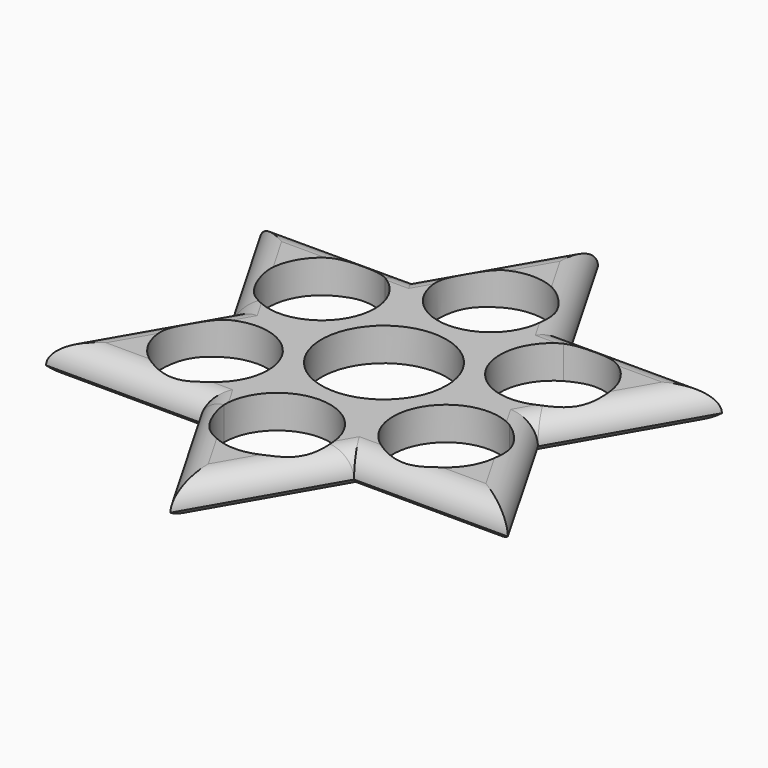
from build123d import *

# Parameters (mm, degrees)
F0_R          = 13.2
F1_DEPTH      = 7
F2_T4_DEPTH   = 57.5870860263
F2_T9_DEPTH   = 57.5217714755
F2_T14_DEPTH  = 57.5217714755
F2_T19_DEPTH  = 57.5870860263
F2_T24_DEPTH  = 57.5870860263
F2_T29_DEPTH  = 57.5217714755
F2_T34_DEPTH  = 57.5217714755
F2_T39_DEPTH  = 57.5870860263
F2_T44_DEPTH  = 57.5870860263
F2_T49_DEPTH  = 57.5217714755
F2_T54_DEPTH  = 57.5217714755
F2_T59_DEPTH  = 57.5870860263
F2_T65_DEPTH  = 57.5870860263
F2_S66_R      = 11.2
F2_T67_DEPTH  = 31
F2_S69_R      = 11.2
F2_T70_DEPTH  = 31
F2_T73_DEPTH  = 57.5870860263
F2_S74_R      = 11.2
F2_T75_DEPTH  = 33
F2_S77_R      = 11.2
F2_T78_DEPTH  = 33
F2_T84_DEPTH  = 57.5217714755
F2_S86_R      = 11.2
F2_T87_DEPTH  = 30
F2_S88_R      = 11.2
F2_T89_DEPTH  = 30
F2_T92_DEPTH  = 57.5217714755
F2_S94_R      = 11.2
F2_T95_DEPTH  = 33
F2_S96_R      = 11.2
F2_T97_DEPTH  = 33
F2_T103_DEPTH = 57.5870860263
F2_S105_R     = 11.2
F2_T106_DEPTH = 33
F2_S107_R     = 11.2
F2_T108_DEPTH = 33
F2_T111_DEPTH = 57.5870860263
F2_S113_R     = 11.2
F2_T114_DEPTH = 33
F2_S115_R     = 11.2
F2_T116_DEPTH = 33
F2_T122_DEPTH = 57.5217714755
F2_S124_R     = 11.2
F2_T125_DEPTH = 33
F2_S126_R     = 11.2
F2_T127_DEPTH = 33
F2_T130_DEPTH = 57.5217714755
F2_S132_R     = 11.2
F2_T133_DEPTH = 30
F2_S134_R     = 11.2
F2_T135_DEPTH = 30
F2_T141_DEPTH = 57.5870860263
F2_S143_R     = 11.2
F2_T144_DEPTH = 31
F2_S145_R     = 11.2
F2_T146_DEPTH = 31
F2_T149_DEPTH = 57.5870860263
F2_S151_R     = 11.2
F2_T152_DEPTH = 33
F2_S153_R     = 11.2
F2_T154_DEPTH = 33
F2_T160_DEPTH = 57.5217714755
F2_S161_R     = 11.2
F2_T162_DEPTH = 33
F2_S164_R     = 11.2
F2_T165_DEPTH = 33
F2_T168_DEPTH = 57.5217714755
F2_S169_R     = 11.2
F2_T170_DEPTH = 33
F2_S172_R     = 11.2
F2_T173_DEPTH = 33
F3_T4_DEPTH   = 52.5217714754
F3_T9_DEPTH   = 52.5870860261
F3_T14_DEPTH  = 52.5870860261
F3_T19_DEPTH  = 52.5217714754
F3_T24_DEPTH  = 52.5217714754
F3_T29_DEPTH  = 52.5870860261
F3_T34_DEPTH  = 52.5870860261
F3_T39_DEPTH  = 52.5217714754
F3_T44_DEPTH  = 52.5217714754
F3_T49_DEPTH  = 52.5870860261
F3_T54_DEPTH  = 52.5217714754
F3_T59_DEPTH  = 52.5870860261
F3_T65_DEPTH  = 52.5217714754
F3_T69_DEPTH  = 52.5217714754
F3_T76_DEPTH  = 52.5870860261
F3_T80_DEPTH  = 52.5870860261
F3_T87_DEPTH  = 52.5217714754
F3_T91_DEPTH  = 52.5217714754
F3_T98_DEPTH  = 52.5870860261
F3_T102_DEPTH = 52.5870860261
F3_T109_DEPTH = 52.5217714754
F3_T113_DEPTH = 52.5217714754
F3_T120_DEPTH = 52.5870860261
F3_T124_DEPTH = 52.5870860261


# Not quite as in the source:
# - a fillet or chamfer that OpenCascade refuses, or shapes differently, is made with other operations: its cross-section is extruded or revolved along the edge and cut away or added


with BuildPart() as f1:
    # F0 (on Top) → F1 (new body)
    with BuildSketch(Plane.XY):
        with BuildLine():
            Line((-16.2445816704, 28.1929764897), (-48.8316676967, 28.1929764897))
            Line((-48.8316676967, 28.1929764897), (-32.5707819589, 0.0282962158))
            Line((-32.5707819589, 0.0282962158), (-30.032715263, 4.4067698189))
            ThreePointArc((-30.032715263, 4.4067698189), (-34.1055736168, 19.7133328412), (-18.7990260705, 23.7862493557))
            Line((-18.7990260705, 23.7862493557), (-16.2445816704, 28.1929764897))
        make_face()
        with BuildLine():
            Line((0.0979717275, 56.3858678653), (-16.2445816704, 28.1929764897))
            Line((-16.2445816704, 28.1929764897), (-11.2, 28.1929764897))
            ThreePointArc((-11.2, 28.1929764897), (0, 39.3929764897), (11.2, 28.1929764897))
            Line((11.2, 28.1929764897), (16.3098962211, 28.1929764897))
            Line((16.3098962211, 28.1929764897), (0.0979717275, 56.3858678653))
        make_face()
        with BuildLine():
            Line((-11.2, 28.1929764897), (-16.2445816704, 28.1929764897))
            Line((-16.2445816704, 28.1929764897), (-18.7990260705, 23.7862493557))
            ThreePointArc((-18.7990260705, 23.7862493557), (-14.7114985514, 19.6880780406), (-13.2158338483, 14.0964882448))
            ThreePointArc((-13.2158338483, 14.0964882448), (-18.8242809265, 4.3921317014), (-30.032715263, 4.4067698189))
            Line((-30.032715263, 4.4067698189), (-32.5707819589, 0.0282962158))
            Line((-32.5707819589, 0.0282962158), (-30.0158338483, -4.3970037224))
            ThreePointArc((-30.0158338483, -4.3970037224), (-18.8158338483, -4.3970037224), (-13.2158338483, -14.0964882448))
            ThreePointArc((-13.2158338483, -14.0964882448), (-14.716349326, -19.6964882448), (-18.8158338483, -23.7959727672))
            Line((-18.8158338483, -23.7959727672), (-16.2935430131, -28.1647086453))
            Line((-16.2935430131, -28.1647086453), (-11.1999831676, -28.1735588213))
            ThreePointArc((-11.1999831676, -28.1735588213), (0.0097088378, -16.9929806978), (11.2, -28.1929764897))
            ThreePointArc((11.2, -28.1929764897), (11.1999957549, -28.2027278845), (11.1999830197, -28.2124792719))
            Line((11.1999830197, -28.2124792719), (16.2608857378, -28.2212727054))
            Line((16.2608857378, -28.2212727054), (18.8158338483, -23.7959727672))
            ThreePointArc((18.8158338483, -23.7959727672), (14.716349326, -8.4964882448), (30.0158338483, -4.3970037224))
            Line((30.0158338483, -4.3970037224), (32.5381246835, -0.0282678444))
            Line((32.5381246835, -0.0282678444), (29.9990092381, 4.3873094656))
            ThreePointArc((29.9990092381, 4.3873094656), (14.7066338546, 8.5133497474), (18.8327322433, 23.805709453))
            Line((18.8327322433, 23.805709453), (16.3098962211, 28.1929764897))
            Line((16.3098962211, 28.1929764897), (11.2, 28.1929764897))
            ThreePointArc((11.2, 28.1929764897), (0, 16.9929764897), (-11.2, 28.1929764897))
        make_face()
        Circle(F0_R, mode=Mode.SUBTRACT)
        with BuildLine():
            Line((-30.0158338483, -4.3970037224), (-32.5707819589, 0.0282962158))
            Line((-32.5707819589, 0.0282962158), (-48.8805798496, -28.1080879278))
            Line((-48.8805798496, -28.1080879278), (-16.2935430131, -28.1647086453))
            Line((-16.2935430131, -28.1647086453), (-18.8158338483, -23.7959727672))
            ThreePointArc((-18.8158338483, -23.7959727672), (-34.1153183707, -19.6964882448), (-30.0158338483, -4.3970037224))
        make_face()
        with BuildLine():
            Line((48.8316676967, 28.1929764897), (16.3098962211, 28.1929764897))
            Line((16.3098962211, 28.1929764897), (18.8327322433, 23.805709453))
            ThreePointArc((18.8327322433, 23.805709453), (30.0242766814, 23.7910933935), (35.6158338483, 14.0964882448))
            ThreePointArc((35.6158338483, 14.0964882448), (34.1104603075, 8.4880822487), (29.9990092381, 4.3873094656))
            Line((29.9990092381, 4.3873094656), (32.5381246835, -0.0282678444))
            Line((32.5381246835, -0.0282678444), (48.8316676967, 28.1929764897))
        make_face()
        with BuildLine():
            Line((-11.1999831676, -28.1735588213), (-16.2935430131, -28.1647086453))
            Line((-16.2935430131, -28.1647086453), (0, -56.3859529793))
            Line((0, -56.3859529793), (16.2608857378, -28.2212727054))
            Line((16.2608857378, -28.2212727054), (11.1999830197, -28.2124792719))
            ThreePointArc((11.1999830197, -28.2124792719), (-0.0194602253, -39.3929595834), (-11.1999831676, -28.1735588213))
        make_face()
        with BuildLine():
            Line((48.7826081221, -28.2777799376), (32.5381246835, -0.0282678444))
            Line((32.5381246835, -0.0282678444), (30.0158338483, -4.3970037224))
            ThreePointArc((30.0158338483, -4.3970037224), (34.1153183707, -8.4964882448), (35.6158338483, -14.0964882448))
            ThreePointArc((35.6158338483, -14.0964882448), (30.0158338483, -23.7959727672), (18.8158338483, -23.7959727672))
            Line((18.8158338483, -23.7959727672), (16.2608857378, -28.2212727054))
            Line((16.2608857378, -28.2212727054), (48.7826081221, -28.2777799376))
        make_face()
    extrude(amount=F1_DEPTH)

    # F2: fillet of radius 5 on 12 edges, made by hand


with BuildPart() as f2_tool2:
    # F2_s3 → F2_t4 (new body)
    with BuildSketch(Plane(origin=(30.7580755612, 53.0614196024, 0), x_dir=(0, 0, 1), z_dir=(-0.5015039818, -0.8651553365, 0))):
        with BuildLine():
            ThreePointArc((2, 28.1929764897), (5.5355339059, 26.7285103956), (7, 23.1929764897))
            Line((7, 23.1929764897), (7, 28.1929764897))
            Line((7, 28.1929764897), (2, 28.1929764897))
        make_face()
    extrude(amount=F2_T4_DEPTH)

    split(bisect_by=Plane.XZ.offset(-28.1929764897), keep=Keep.BOTTOM)


with BuildPart() as f1_1:
    add(f1.part)

    # F2_t1: cut F2_tool2
    add(f2_tool2.part, mode=Mode.SUBTRACT)


with BuildPart() as f2_tool7:
    # F2_s8 → F2_t9 (new body)
    with BuildSketch(Plane(origin=(-1.8992123449, 3.3027718184, 0), x_dir=(0, 0, 1), z_dir=(-0.4984945087, 0.8668928566, 0))):
        with BuildLine():
            ThreePointArc((2, 28.1929764897), (5.5355339059, 26.7285103956), (7, 23.1929764897))
            Line((7, 23.1929764897), (7, 28.1929764897))
            Line((7, 28.1929764897), (2, 28.1929764897))
        make_face()
    extrude(amount=F2_T9_DEPTH)

    split(bisect_by=Plane.XZ.offset(-28.1929764897), keep=Keep.BOTTOM)


with BuildPart() as f1_2:
    add(f1_1.part)

    # F2_t6: cut F2_tool7
    add(f2_tool7.part, mode=Mode.SUBTRACT)


with BuildPart() as f2_tool12:
    # F2_s13 → F2_t14 (new body)
    with BuildSketch(Plane.YZ.offset(61.3316676967)):
        with BuildLine():
            ThreePointArc((28.1929764897, 2), (26.7285103956, 5.5355339059), (23.1929764897, 7))
            Line((23.1929764897, 7), (28.1929764897, 7))
            Line((28.1929764897, 7), (28.1929764897, 2))
        make_face()
    extrude(amount=-F2_T14_DEPTH)

    split(bisect_by=Plane(origin=(24.4402899248, 14.0540439639, 0), x_dir=(0, 0, 1), z_dir=(0.8668928566, 0.4984945087, 0)), keep=Keep.TOP)


with BuildPart() as f1_3:
    add(f1_2.part)

    # F2_t11: cut F2_tool12
    add(f2_tool12.part, mode=Mode.SUBTRACT)


with BuildPart() as f2_tool17:
    # F2_s18 → F2_t19 (new body)
    with BuildSketch(Plane(origin=(1.8722908352, 3.2429028531, 0), x_dir=(0, 0, 1), z_dir=(0.5, 0.8660254038, 0))):
        with BuildLine():
            ThreePointArc((2, 28.1929764897), (5.5355339059, 26.7285103956), (7, 23.1929764897))
            Line((7, 23.1929764897), (7, 28.1929764897))
            Line((7, 28.1929764897), (2, 28.1929764897))
        make_face()
    extrude(amount=F2_T19_DEPTH)

    split(bisect_by=Plane(origin=(24.4402899248, 14.0540439639, 0), x_dir=(0, 0, 1), z_dir=(0.8668928566, 0.4984945087, 0)), keep=Keep.TOP)


with BuildPart() as f1_4:
    add(f1_3.part)

    # F2_t16: cut F2_tool17
    add(f2_tool17.part, mode=Mode.SUBTRACT)


with BuildPart() as f2_tool22:
    # F2_s23 → F2_t24 (new body)
    with BuildSketch(Plane(origin=(30.573499556, -53.1679846088, 0), x_dir=(0, 0, 1), z_dir=(-0.4984945087, 0.8668928566, 0))):
        with BuildLine():
            ThreePointArc((2, 28.1929764897), (5.5355339059, 26.7285103956), (7, 23.1929764897))
            Line((7, 23.1929764897), (7, 28.1929764897))
            Line((7, 28.1929764897), (2, 28.1929764897))
        make_face()
    extrude(amount=F2_T24_DEPTH)

    split(bisect_by=Plane(origin=(24.4158338483, -14.0964882448, 0), x_dir=(0, 0, 1), z_dir=(0.8660254038, -0.5, 0)), keep=Keep.TOP)


with BuildPart() as f1_5:
    add(f1_4.part)

    # F2_t21: cut F2_tool22
    add(f2_tool22.part, mode=Mode.SUBTRACT)


with BuildPart() as f2_tool27:
    # F2_s28 → F2_t29 (new body)
    with BuildSketch(Plane(origin=(3.8098904701, -0.0066197713, 0), x_dir=(0, 0, 1), z_dir=(0.9999984905, -0.0017375201, 0))):
        with BuildLine():
            ThreePointArc((2, 28.1929764897), (5.5355339059, 26.7285103956), (7, 23.1929764897))
            Line((7, 23.1929764897), (7, 28.1929764897))
            Line((7, 28.1929764897), (2, 28.1929764897))
        make_face()
    extrude(amount=F2_T29_DEPTH)

    split(bisect_by=Plane(origin=(24.4158338483, -14.0964882448, 0), x_dir=(0, 0, 1), z_dir=(0.8660254038, -0.5, 0)), keep=Keep.TOP)


with BuildPart() as f1_6:
    add(f1_5.part)

    # F2_t26: cut F2_tool27
    add(f2_tool27.part, mode=Mode.SUBTRACT)


with BuildPart() as f2_tool32:
    # F2_s33 → F2_t34 (new body)
    with BuildSketch(Plane(origin=(-30.6658338483, -53.1147822818, 0), x_dir=(0, 0, 1), z_dir=(0.5, 0.8660254038, 0))):
        with BuildLine():
            ThreePointArc((2, 28.1929764897), (5.5355339059, 26.7285103956), (7, 23.1929764897))
            Line((7, 23.1929764897), (7, 28.1929764897))
            Line((7, 28.1929764897), (2, 28.1929764897))
        make_face()
    extrude(amount=F2_T34_DEPTH)

    split(bisect_by=Plane(origin=(-0.0489858638, -28.1929339327, 0), x_dir=(0, 0, 1), z_dir=(-0.0017375201, -0.9999984905, 0)), keep=Keep.TOP)


with BuildPart() as f1_7:
    add(f1_6.part)

    # F2_t31: cut F2_tool32
    add(f2_tool32.part, mode=Mode.SUBTRACT)


with BuildPart() as f2_tool37:
    # F2_s38 → F2_t39 (new body)
    with BuildSketch(Plane(origin=(1.8722908352, -3.2429028531, 0), x_dir=(0, 0, 1), z_dir=(0.5, -0.8660254038, 0))):
        with BuildLine():
            ThreePointArc((2, 28.1929764897), (5.5355339059, 26.7285103956), (7, 23.1929764897))
            Line((7, 23.1929764897), (7, 28.1929764897))
            Line((7, 28.1929764897), (2, 28.1929764897))
        make_face()
    extrude(amount=F2_T39_DEPTH)

    split(bisect_by=Plane(origin=(-0.0489858638, -28.1929339327, 0), x_dir=(0, 0, 1), z_dir=(-0.0017375201, -0.9999984905, 0)), keep=Keep.TOP)


with BuildPart() as f1_8:
    add(f1_7.part)

    # F2_t36: cut F2_tool37
    add(f2_tool37.part, mode=Mode.SUBTRACT)


with BuildPart() as f2_tool42:
    # F2_s43 → F2_t44 (new body)
    with BuildSketch(Plane(origin=(-61.3315751172, 0.1065650063, 0), x_dir=(0, 0, 1), z_dir=(0.9999984905, -0.0017375201, 0))):
        with BuildLine():
            ThreePointArc((2, 28.1929764897), (5.5355339059, 26.7285103956), (7, 23.1929764897))
            Line((7, 23.1929764897), (7, 28.1929764897))
            Line((7, 28.1929764897), (2, 28.1929764897))
        make_face()
    extrude(amount=F2_T44_DEPTH)

    split(bisect_by=Plane(origin=(-24.4158338483, -14.0964882448, 0), x_dir=(0, 0, 1), z_dir=(-0.8660254038, -0.5, 0)), keep=Keep.TOP)


with BuildPart() as f1_9:
    add(f1_8.part)

    # F2_t41: cut F2_tool42
    add(f2_tool42.part, mode=Mode.SUBTRACT)


with BuildPart() as f2_tool47:
    # F2_s48 → F2_t49 (new body)
    with BuildSketch(Plane(origin=(-1.9106781252, -3.2961520471, 0), x_dir=(0, 0, 1), z_dir=(-0.5015039818, -0.8651553365, 0))):
        with BuildLine():
            ThreePointArc((2, 28.1929764897), (5.5355339059, 26.7285103956), (7, 23.1929764897))
            Line((7, 23.1929764897), (7, 28.1929764897))
            Line((7, 28.1929764897), (2, 28.1929764897))
        make_face()
    extrude(amount=F2_T49_DEPTH)

    split(bisect_by=Plane(origin=(-24.4158338483, -14.0964882448, 0), x_dir=(0, 0, 1), z_dir=(-0.8660254038, -0.5, 0)), keep=Keep.TOP)


with BuildPart() as f1_10:
    add(f1_9.part)

    # F2_t46: cut F2_tool47
    add(f2_tool47.part, mode=Mode.SUBTRACT)


with BuildPart() as f2_tool52:
    # F2_s53 → F2_t54 (new body)
    with BuildSketch(Plane(origin=(-30.6658338483, 53.1147822818, 0), x_dir=(0, 0, 1), z_dir=(0.5, -0.8660254038, 0))):
        with BuildLine():
            ThreePointArc((2, 28.1929764897), (5.5355339059, 26.7285103956), (7, 23.1929764897))
            Line((7, 23.1929764897), (7, 28.1929764897))
            Line((7, 28.1929764897), (2, 28.1929764897))
        make_face()
    extrude(amount=F2_T54_DEPTH)

    split(bisect_by=Plane(origin=(-24.391304061, 14.1388899688, 0), x_dir=(0, 0, 1), z_dir=(-0.8651553365, 0.5015039818, 0)), keep=Keep.TOP)


with BuildPart() as f1_11:
    add(f1_10.part)

    # F2_t51: cut F2_tool52
    add(f2_tool52.part, mode=Mode.SUBTRACT)


with BuildPart() as f2_tool57:
    # F2_s58 → F2_t59 (new body)
    with BuildSketch(Plane.YZ.offset(-3.7445816704)):
        with BuildLine():
            ThreePointArc((28.1929764897, 2), (26.7285103956, 5.5355339059), (23.1929764897, 7))
            Line((23.1929764897, 7), (28.1929764897, 7))
            Line((28.1929764897, 7), (28.1929764897, 2))
        make_face()
    extrude(amount=-F2_T59_DEPTH)

    split(bisect_by=Plane(origin=(-24.391304061, 14.1388899688, 0), x_dir=(0, 0, 1), z_dir=(-0.8651553365, 0.5015039818, 0)), keep=Keep.TOP)


with BuildPart() as f1_12:
    add(f1_11.part)

    # F2_t56: cut F2_tool57
    add(f2_tool57.part, mode=Mode.SUBTRACT)


with BuildPart() as f2_tool63:
    # F2_s64 → F2_t65 (new body)
    with BuildSketch(Plane.YZ.offset(-3.7445816704)):
        with BuildLine():
            ThreePointArc((28.1929764897, 2), (26.7285103956, 5.5355339059), (23.1929764897, 7))
            Line((23.1929764897, 7), (28.1929764897, 7))
            Line((28.1929764897, 7), (28.1929764897, 2))
        make_face()
    extrude(amount=-F2_T65_DEPTH)

    # F2_s66 → F2_t67 (cut, symmetric)
    with BuildSketch(Plane.XY.offset(4.5)):
        with Locations((-24.4158338483, 14.0964882448)):
            Circle(F2_S66_R)
    extrude(amount=F2_T67_DEPTH, both=True, mode=Mode.SUBTRACT)

    split(bisect_by=Plane(origin=(-24.391304061, 14.1388899688, 0), x_dir=(0, 0, 1), z_dir=(0.8651553365, -0.5015039818, 0)), keep=Keep.TOP)

    # F2_s69 → F2_t70 (cut, symmetric)
    with BuildSketch(Plane.XY.offset(4.5)):
        with Locations((0, 28.1929764897)):
            Circle(F2_S69_R)
    extrude(amount=F2_T70_DEPTH, both=True, mode=Mode.SUBTRACT)


with BuildPart() as f2_tool71:
    # F2_s72 → F2_t73 (new body)
    with BuildSketch(Plane(origin=(30.7580755612, 53.0614196024, 0), x_dir=(0, 0, 1), z_dir=(-0.5015039818, -0.8651553365, 0))):
        with BuildLine():
            ThreePointArc((2, 28.1929764897), (5.5355339059, 26.7285103956), (7, 23.1929764897))
            Line((7, 23.1929764897), (7, 28.1929764897))
            Line((7, 28.1929764897), (2, 28.1929764897))
        make_face()
    extrude(amount=F2_T73_DEPTH)

    # F2_s74 → F2_t75 (cut, symmetric)
    with BuildSketch(Plane.XY.offset(4.5)):
        with Locations((-24.4158338483, 14.0964882448)):
            Circle(F2_S74_R)
    extrude(amount=F2_T75_DEPTH, both=True, mode=Mode.SUBTRACT)

    split(bisect_by=Plane.XZ.offset(-28.1929764897), keep=Keep.TOP)

    # F2_s77 → F2_t78 (cut, symmetric)
    with BuildSketch(Plane.XY.offset(4.5)):
        with Locations((0, 28.1929764897)):
            Circle(F2_S77_R)
    extrude(amount=F2_T78_DEPTH, both=True, mode=Mode.SUBTRACT)


with BuildPart() as f2_tool63_1:
    add(f2_tool63.part)

    # F2_t79: intersect F2_tool71
    add(f2_tool71.part, mode=Mode.INTERSECT)


with BuildPart() as f1_13:
    add(f1_12.part)

    # F2_t61: cut F2_tool63
    add(f2_tool63_1.part, mode=Mode.SUBTRACT)


with BuildPart() as f2_tool82:
    # F2_s83 → F2_t84 (new body)
    with BuildSketch(Plane.YZ.offset(61.3316676967)):
        with BuildLine():
            ThreePointArc((28.1929764897, 2), (26.7285103956, 5.5355339059), (23.1929764897, 7))
            Line((23.1929764897, 7), (28.1929764897, 7))
            Line((28.1929764897, 7), (28.1929764897, 2))
        make_face()
    extrude(amount=-F2_T84_DEPTH)

    split(bisect_by=Plane(origin=(24.4402899248, 14.0540439639, 0), x_dir=(0, 0, 1), z_dir=(-0.8668928566, -0.4984945087, 0)), keep=Keep.TOP)

    # F2_s86 → F2_t87 (cut, symmetric)
    with BuildSketch(Plane.XY.offset(4.5)):
        with Locations((24.4158338483, 14.0964882448)):
            Circle(F2_S86_R)
    extrude(amount=F2_T87_DEPTH, both=True, mode=Mode.SUBTRACT)

    # F2_s88 → F2_t89 (cut, symmetric)
    with BuildSketch(Plane.XY.offset(4.5)):
        with Locations((0, 28.1929764897)):
            Circle(F2_S88_R)
    extrude(amount=F2_T89_DEPTH, both=True, mode=Mode.SUBTRACT)


with BuildPart() as f2_tool90:
    # F2_s91 → F2_t92 (new body)
    with BuildSketch(Plane(origin=(-1.8992123449, 3.3027718184, 0), x_dir=(0, 0, 1), z_dir=(-0.4984945087, 0.8668928566, 0))):
        with BuildLine():
            ThreePointArc((2, 28.1929764897), (5.5355339059, 26.7285103956), (7, 23.1929764897))
            Line((7, 23.1929764897), (7, 28.1929764897))
            Line((7, 28.1929764897), (2, 28.1929764897))
        make_face()
    extrude(amount=F2_T92_DEPTH)

    split(bisect_by=Plane.XZ.offset(-28.1929764897), keep=Keep.TOP)

    # F2_s94 → F2_t95 (cut, symmetric)
    with BuildSketch(Plane.XY.offset(4.5)):
        with Locations((24.4158338483, 14.0964882448)):
            Circle(F2_S94_R)
    extrude(amount=F2_T95_DEPTH, both=True, mode=Mode.SUBTRACT)

    # F2_s96 → F2_t97 (cut, symmetric)
    with BuildSketch(Plane.XY.offset(4.5)):
        with Locations((0, 28.1929764897)):
            Circle(F2_S96_R)
    extrude(amount=F2_T97_DEPTH, both=True, mode=Mode.SUBTRACT)


with BuildPart() as f2_tool82_1:
    add(f2_tool82.part)

    # F2_t98: intersect F2_tool90
    add(f2_tool90.part, mode=Mode.INTERSECT)


with BuildPart() as f1_14:
    add(f1_13.part)

    # F2_t80: cut F2_tool82
    add(f2_tool82_1.part, mode=Mode.SUBTRACT)


with BuildPart() as f2_tool101:
    # F2_s102 → F2_t103 (new body)
    with BuildSketch(Plane(origin=(30.573499556, -53.1679846088, 0), x_dir=(0, 0, 1), z_dir=(-0.4984945087, 0.8668928566, 0))):
        with BuildLine():
            ThreePointArc((2, 28.1929764897), (5.5355339059, 26.7285103956), (7, 23.1929764897))
            Line((7, 23.1929764897), (7, 28.1929764897))
            Line((7, 28.1929764897), (2, 28.1929764897))
        make_face()
    extrude(amount=F2_T103_DEPTH)

    split(bisect_by=Plane(origin=(24.4158338483, -14.0964882448, 0), x_dir=(0, 0, 1), z_dir=(-0.8660254038, 0.5, 0)), keep=Keep.TOP)

    # F2_s105 → F2_t106 (cut, symmetric)
    with BuildSketch(Plane.XY.offset(4.5)):
        with Locations((24.4158338483, -14.0964882448)):
            Circle(F2_S105_R)
    extrude(amount=F2_T106_DEPTH, both=True, mode=Mode.SUBTRACT)

    # F2_s107 → F2_t108 (cut, symmetric)
    with BuildSketch(Plane.XY.offset(4.5)):
        with Locations((24.4158338483, 14.0964882448)):
            Circle(F2_S107_R)
    extrude(amount=F2_T108_DEPTH, both=True, mode=Mode.SUBTRACT)


with BuildPart() as f2_tool109:
    # F2_s110 → F2_t111 (new body)
    with BuildSketch(Plane(origin=(1.8722908352, 3.2429028531, 0), x_dir=(0, 0, 1), z_dir=(0.5, 0.8660254038, 0))):
        with BuildLine():
            ThreePointArc((2, 28.1929764897), (5.5355339059, 26.7285103956), (7, 23.1929764897))
            Line((7, 23.1929764897), (7, 28.1929764897))
            Line((7, 28.1929764897), (2, 28.1929764897))
        make_face()
    extrude(amount=F2_T111_DEPTH)

    split(bisect_by=Plane(origin=(24.4402899248, 14.0540439639, 0), x_dir=(0, 0, 1), z_dir=(-0.8668928566, -0.4984945087, 0)), keep=Keep.TOP)

    # F2_s113 → F2_t114 (cut, symmetric)
    with BuildSketch(Plane.XY.offset(4.5)):
        with Locations((24.4158338483, -14.0964882448)):
            Circle(F2_S113_R)
    extrude(amount=F2_T114_DEPTH, both=True, mode=Mode.SUBTRACT)

    # F2_s115 → F2_t116 (cut, symmetric)
    with BuildSketch(Plane.XY.offset(4.5)):
        with Locations((24.4158338483, 14.0964882448)):
            Circle(F2_S115_R)
    extrude(amount=F2_T116_DEPTH, both=True, mode=Mode.SUBTRACT)


with BuildPart() as f2_tool101_1:
    add(f2_tool101.part)

    # F2_t117: intersect F2_tool109
    add(f2_tool109.part, mode=Mode.INTERSECT)


with BuildPart() as f1_15:
    add(f1_14.part)

    # F2_t99: cut F2_tool101
    add(f2_tool101_1.part, mode=Mode.SUBTRACT)


with BuildPart() as f2_tool120:
    # F2_s121 → F2_t122 (new body)
    with BuildSketch(Plane(origin=(-30.6658338483, -53.1147822818, 0), x_dir=(0, 0, 1), z_dir=(0.5, 0.8660254038, 0))):
        with BuildLine():
            ThreePointArc((2, 28.1929764897), (5.5355339059, 26.7285103956), (7, 23.1929764897))
            Line((7, 23.1929764897), (7, 28.1929764897))
            Line((7, 28.1929764897), (2, 28.1929764897))
        make_face()
    extrude(amount=F2_T122_DEPTH)

    split(bisect_by=Plane(origin=(-0.0489858638, -28.1929339327, 0), x_dir=(0, 0, 1), z_dir=(0.0017375201, 0.9999984905, 0)), keep=Keep.TOP)

    # F2_s124 → F2_t125 (cut, symmetric)
    with BuildSketch(Plane.XY.offset(4.5)):
        with Locations((24.4158338483, -14.0964882448)):
            Circle(F2_S124_R)
    extrude(amount=F2_T125_DEPTH, both=True, mode=Mode.SUBTRACT)

    # F2_s126 → F2_t127 (cut, symmetric)
    with BuildSketch(Plane.XY.offset(4.5)):
        with Locations((0, -28.1929764897)):
            Circle(F2_S126_R)
    extrude(amount=F2_T127_DEPTH, both=True, mode=Mode.SUBTRACT)


with BuildPart() as f2_tool128:
    # F2_s129 → F2_t130 (new body)
    with BuildSketch(Plane(origin=(3.8098904701, -0.0066197713, 0), x_dir=(0, 0, 1), z_dir=(0.9999984905, -0.0017375201, 0))):
        with BuildLine():
            ThreePointArc((2, 28.1929764897), (5.5355339059, 26.7285103956), (7, 23.1929764897))
            Line((7, 23.1929764897), (7, 28.1929764897))
            Line((7, 28.1929764897), (2, 28.1929764897))
        make_face()
    extrude(amount=F2_T130_DEPTH)

    split(bisect_by=Plane(origin=(24.4158338483, -14.0964882448, 0), x_dir=(0, 0, 1), z_dir=(-0.8660254038, 0.5, 0)), keep=Keep.TOP)

    # F2_s132 → F2_t133 (cut, symmetric)
    with BuildSketch(Plane.XY.offset(4.5)):
        with Locations((24.4158338483, -14.0964882448)):
            Circle(F2_S132_R)
    extrude(amount=F2_T133_DEPTH, both=True, mode=Mode.SUBTRACT)

    # F2_s134 → F2_t135 (cut, symmetric)
    with BuildSketch(Plane.XY.offset(4.5)):
        with Locations((0, -28.1929764897)):
            Circle(F2_S134_R)
    extrude(amount=F2_T135_DEPTH, both=True, mode=Mode.SUBTRACT)


with BuildPart() as f2_tool120_1:
    add(f2_tool120.part)

    # F2_t136: intersect F2_tool128
    add(f2_tool128.part, mode=Mode.INTERSECT)


with BuildPart() as f1_16:
    add(f1_15.part)

    # F2_t118: cut F2_tool120
    add(f2_tool120_1.part, mode=Mode.SUBTRACT)


with BuildPart() as f2_tool139:
    # F2_s140 → F2_t141 (new body)
    with BuildSketch(Plane(origin=(-61.3315751172, 0.1065650063, 0), x_dir=(0, 0, 1), z_dir=(0.9999984905, -0.0017375201, 0))):
        with BuildLine():
            ThreePointArc((2, 28.1929764897), (5.5355339059, 26.7285103956), (7, 23.1929764897))
            Line((7, 23.1929764897), (7, 28.1929764897))
            Line((7, 28.1929764897), (2, 28.1929764897))
        make_face()
    extrude(amount=F2_T141_DEPTH)

    split(bisect_by=Plane(origin=(-24.4158338483, -14.0964882448, 0), x_dir=(0, 0, 1), z_dir=(0.8660254038, 0.5, 0)), keep=Keep.TOP)

    # F2_s143 → F2_t144 (cut, symmetric)
    with BuildSketch(Plane.XY.offset(4.5)):
        with Locations((0, -28.1929764897)):
            Circle(F2_S143_R)
    extrude(amount=F2_T144_DEPTH, both=True, mode=Mode.SUBTRACT)

    # F2_s145 → F2_t146 (cut, symmetric)
    with BuildSketch(Plane.XY.offset(4.5)):
        with Locations((-24.4158338483, -14.0964882448)):
            Circle(F2_S145_R)
    extrude(amount=F2_T146_DEPTH, both=True, mode=Mode.SUBTRACT)


with BuildPart() as f2_tool147:
    # F2_s148 → F2_t149 (new body)
    with BuildSketch(Plane(origin=(1.8722908352, -3.2429028531, 0), x_dir=(0, 0, 1), z_dir=(0.5, -0.8660254038, 0))):
        with BuildLine():
            ThreePointArc((2, 28.1929764897), (5.5355339059, 26.7285103956), (7, 23.1929764897))
            Line((7, 23.1929764897), (7, 28.1929764897))
            Line((7, 28.1929764897), (2, 28.1929764897))
        make_face()
    extrude(amount=F2_T149_DEPTH)

    split(bisect_by=Plane(origin=(-0.0489858638, -28.1929339327, 0), x_dir=(0, 0, 1), z_dir=(0.0017375201, 0.9999984905, 0)), keep=Keep.TOP)

    # F2_s151 → F2_t152 (cut, symmetric)
    with BuildSketch(Plane.XY.offset(4.5)):
        with Locations((0, -28.1929764897)):
            Circle(F2_S151_R)
    extrude(amount=F2_T152_DEPTH, both=True, mode=Mode.SUBTRACT)

    # F2_s153 → F2_t154 (cut, symmetric)
    with BuildSketch(Plane.XY.offset(4.5)):
        with Locations((-24.4158338483, -14.0964882448)):
            Circle(F2_S153_R)
    extrude(amount=F2_T154_DEPTH, both=True, mode=Mode.SUBTRACT)


with BuildPart() as f2_tool139_1:
    add(f2_tool139.part)

    # F2_t155: intersect F2_tool147
    add(f2_tool147.part, mode=Mode.INTERSECT)


with BuildPart() as f1_17:
    add(f1_16.part)

    # F2_t137: cut F2_tool139
    add(f2_tool139_1.part, mode=Mode.SUBTRACT)


with BuildPart() as f2_tool158:
    # F2_s159 → F2_t160 (new body)
    with BuildSketch(Plane(origin=(-30.6658338483, 53.1147822818, 0), x_dir=(0, 0, 1), z_dir=(0.5, -0.8660254038, 0))):
        with BuildLine():
            ThreePointArc((2, 28.1929764897), (5.5355339059, 26.7285103956), (7, 23.1929764897))
            Line((7, 23.1929764897), (7, 28.1929764897))
            Line((7, 28.1929764897), (2, 28.1929764897))
        make_face()
    extrude(amount=F2_T160_DEPTH)

    # F2_s161 → F2_t162 (cut, symmetric)
    with BuildSketch(Plane.XY.offset(4.5)):
        with Locations((-24.4158338483, 14.0964882448)):
            Circle(F2_S161_R)
    extrude(amount=F2_T162_DEPTH, both=True, mode=Mode.SUBTRACT)

    split(bisect_by=Plane(origin=(-24.391304061, 14.1388899688, 0), x_dir=(0, 0, 1), z_dir=(0.8651553365, -0.5015039818, 0)), keep=Keep.TOP)

    # F2_s164 → F2_t165 (cut, symmetric)
    with BuildSketch(Plane.XY.offset(4.5)):
        with Locations((-24.4158338483, -14.0964882448)):
            Circle(F2_S164_R)
    extrude(amount=F2_T165_DEPTH, both=True, mode=Mode.SUBTRACT)


with BuildPart() as f2_tool166:
    # F2_s167 → F2_t168 (new body)
    with BuildSketch(Plane(origin=(-1.9106781252, -3.2961520471, 0), x_dir=(0, 0, 1), z_dir=(-0.5015039818, -0.8651553365, 0))):
        with BuildLine():
            ThreePointArc((2, 28.1929764897), (5.5355339059, 26.7285103956), (7, 23.1929764897))
            Line((7, 23.1929764897), (7, 28.1929764897))
            Line((7, 28.1929764897), (2, 28.1929764897))
        make_face()
    extrude(amount=F2_T168_DEPTH)

    # F2_s169 → F2_t170 (cut, symmetric)
    with BuildSketch(Plane.XY.offset(4.5)):
        with Locations((-24.4158338483, 14.0964882448)):
            Circle(F2_S169_R)
    extrude(amount=F2_T170_DEPTH, both=True, mode=Mode.SUBTRACT)

    split(bisect_by=Plane(origin=(-24.4158338483, -14.0964882448, 0), x_dir=(0, 0, 1), z_dir=(0.8660254038, 0.5, 0)), keep=Keep.TOP)

    # F2_s172 → F2_t173 (cut, symmetric)
    with BuildSketch(Plane.XY.offset(4.5)):
        with Locations((-24.4158338483, -14.0964882448)):
            Circle(F2_S172_R)
    extrude(amount=F2_T173_DEPTH, both=True, mode=Mode.SUBTRACT)


with BuildPart() as f2_tool158_1:
    add(f2_tool158.part)

    # F2_t174: intersect F2_tool166
    add(f2_tool166.part, mode=Mode.INTERSECT)


with BuildPart() as f1_18:
    add(f1_17.part)

    # F2_t156: cut F2_tool158
    add(f2_tool158_1.part, mode=Mode.SUBTRACT)

    # F3: fillet of radius 5 on 12 edges, made by hand


with BuildPart() as f3_tool2:
    # F3_s3 → F3_t4 (new body)
    with BuildSketch(Plane.YZ.offset(58.8316676966)):
        with BuildLine():
            ThreePointArc((24.1929764897, 0), (26.4290444672, 0.527864045), (28.1929764897, 2))
            Line((28.1929764897, 2), (28.2729764897, 1.94))
            ThreePointArc((28.2729764897, 1.94), (28.2929764897, 1), (28.2929764897, 0))
            Line((28.2929764897, 0), (28.1929764897, -0.1))
            Line((28.1929764897, -0.1), (24.1929764897, -0.1))
            Line((24.1929764897, -0.1), (24.1929764897, 0))
        make_face()
    extrude(amount=-F3_T4_DEPTH)

    split(bisect_by=Plane(origin=(24.4402899248, 14.0540439639, 0), x_dir=(0, 0, 1), z_dir=(0.8668928566, 0.4984945087, 0)), keep=Keep.TOP)


with BuildPart() as f1_19:
    add(f1_18.part)

    # F3_t1: cut F3_tool2
    add(f3_tool2.part, mode=Mode.SUBTRACT)


with BuildPart() as f3_tool7:
    # F3_s8 → F3_t9 (new body)
    with BuildSketch(Plane(origin=(3.1222908352, 5.4079663627, 0), x_dir=(0, 0, 1), z_dir=(0.5, 0.8660254038, 0))):
        with BuildLine():
            ThreePointArc((0, 24.1929764897), (0.527864045, 26.4290444672), (2, 28.1929764897))
            Line((2, 28.1929764897), (1.94, 28.2729764897))
            ThreePointArc((1.94, 28.2729764897), (1, 28.2929764897), (0, 28.2929764897))
            Line((0, 28.2929764897), (-0.1, 28.1929764897))
            Line((-0.1, 28.1929764897), (-0.1, 24.1929764897))
            Line((-0.1, 24.1929764897), (0, 24.1929764897))
        make_face()
    extrude(amount=F3_T9_DEPTH)

    split(bisect_by=Plane(origin=(24.4402899248, 14.0540439639, 0), x_dir=(0, 0, 1), z_dir=(0.8668928566, 0.4984945087, 0)), keep=Keep.TOP)


with BuildPart() as f1_20:
    add(f1_19.part)

    # F3_t6: cut F3_tool7
    add(f3_tool7.part, mode=Mode.SUBTRACT)


with BuildPart() as f3_tool12:
    # F3_s13 → F3_t14 (new body)
    with BuildSketch(Plane(origin=(29.3272632842, -51.0007524672, 0), x_dir=(0, 0, 1), z_dir=(-0.4984945087, 0.8668928566, 0))):
        with BuildLine():
            ThreePointArc((0, 24.1929764897), (0.527864045, 26.4290444672), (2, 28.1929764897))
            Line((2, 28.1929764897), (1.94, 28.2729764897))
            ThreePointArc((1.94, 28.2729764897), (1, 28.2929764897), (0, 28.2929764897))
            Line((0, 28.2929764897), (-0.1, 28.1929764897))
            Line((-0.1, 28.1929764897), (-0.1, 24.1929764897))
            Line((-0.1, 24.1929764897), (0, 24.1929764897))
        make_face()
    extrude(amount=F3_T14_DEPTH)

    split(bisect_by=Plane(origin=(24.4158338483, -14.0964882448, 0), x_dir=(0, 0, 1), z_dir=(0.8660254038, -0.5, 0)), keep=Keep.TOP)


with BuildPart() as f1_21:
    add(f1_20.part)

    # F3_t11: cut F3_tool12
    add(f3_tool12.part, mode=Mode.SUBTRACT)


with BuildPart() as f3_tool17:
    # F3_s18 → F3_t19 (new body)
    with BuildSketch(Plane(origin=(6.3098866965, -0.0109635716, 0), x_dir=(0, 0, 1), z_dir=(0.9999984905, -0.0017375201, 0))):
        with BuildLine():
            ThreePointArc((0, 24.1929764897), (0.527864045, 26.4290444672), (2, 28.1929764897))
            Line((2, 28.1929764897), (1.94, 28.2729764897))
            ThreePointArc((1.94, 28.2729764897), (1, 28.2929764897), (0, 28.2929764897))
            Line((0, 28.2929764897), (-0.1, 28.1929764897))
            Line((-0.1, 28.1929764897), (-0.1, 24.1929764897))
            Line((-0.1, 24.1929764897), (0, 24.1929764897))
        make_face()
    extrude(amount=F3_T19_DEPTH)

    split(bisect_by=Plane(origin=(24.4158338483, -14.0964882448, 0), x_dir=(0, 0, 1), z_dir=(0.8660254038, -0.5, 0)), keep=Keep.TOP)


with BuildPart() as f1_22:
    add(f1_21.part)

    # F3_t16: cut F3_tool17
    add(f3_tool17.part, mode=Mode.SUBTRACT)


with BuildPart() as f3_tool22:
    # F3_s23 → F3_t24 (new body)
    with BuildSketch(Plane(origin=(-29.4158338483, -50.9497187723, 0), x_dir=(0, 0, 1), z_dir=(0.5, 0.8660254038, 0))):
        with BuildLine():
            ThreePointArc((0, 24.1929764897), (0.527864045, 26.4290444672), (2, 28.1929764897))
            Line((2, 28.1929764897), (1.94, 28.2729764897))
            ThreePointArc((1.94, 28.2729764897), (1, 28.2929764897), (0, 28.2929764897))
            Line((0, 28.2929764897), (-0.1, 28.1929764897))
            Line((-0.1, 28.1929764897), (-0.1, 24.1929764897))
            Line((-0.1, 24.1929764897), (0, 24.1929764897))
        make_face()
    extrude(amount=F3_T24_DEPTH)

    split(bisect_by=Plane(origin=(-0.0489858638, -28.1929339327, 0), x_dir=(0, 0, 1), z_dir=(-0.0017375201, -0.9999984905, 0)), keep=Keep.TOP)


with BuildPart() as f1_23:
    add(f1_22.part)

    # F3_t21: cut F3_tool22
    add(f3_tool22.part, mode=Mode.SUBTRACT)


with BuildPart() as f3_tool27:
    # F3_s28 → F3_t29 (new body)
    with BuildSketch(Plane(origin=(3.1222908352, -5.4079663627, 0), x_dir=(0, 0, 1), z_dir=(0.5, -0.8660254038, 0))):
        with BuildLine():
            ThreePointArc((0, 24.1929764897), (0.527864045, 26.4290444672), (2, 28.1929764897))
            Line((2, 28.1929764897), (1.94, 28.2729764897))
            ThreePointArc((1.94, 28.2729764897), (1, 28.2929764897), (0, 28.2929764897))
            Line((0, 28.2929764897), (-0.1, 28.1929764897))
            Line((-0.1, 28.1929764897), (-0.1, 24.1929764897))
            Line((-0.1, 24.1929764897), (0, 24.1929764897))
        make_face()
    extrude(amount=F3_T29_DEPTH)

    split(bisect_by=Plane(origin=(-0.0489858638, -28.1929339327, 0), x_dir=(0, 0, 1), z_dir=(-0.0017375201, -0.9999984905, 0)), keep=Keep.TOP)


with BuildPart() as f1_24:
    add(f1_23.part)

    # F3_t26: cut F3_tool27
    add(f3_tool27.part, mode=Mode.SUBTRACT)


with BuildPart() as f3_tool32:
    # F3_s33 → F3_t34 (new body)
    with BuildSketch(Plane(origin=(-58.8315788908, 0.102221206, 0), x_dir=(0, 0, 1), z_dir=(0.9999984905, -0.0017375201, 0))):
        with BuildLine():
            ThreePointArc((0, 24.1929764897), (0.527864045, 26.4290444672), (2, 28.1929764897))
            Line((2, 28.1929764897), (1.94, 28.2729764897))
            ThreePointArc((1.94, 28.2729764897), (1, 28.2929764897), (0, 28.2929764897))
            Line((0, 28.2929764897), (-0.1, 28.1929764897))
            Line((-0.1, 28.1929764897), (-0.1, 24.1929764897))
            Line((-0.1, 24.1929764897), (0, 24.1929764897))
        make_face()
    extrude(amount=F3_T34_DEPTH)

    split(bisect_by=Plane(origin=(-24.4158338483, -14.0964882448, 0), x_dir=(0, 0, 1), z_dir=(-0.8660254038, -0.5, 0)), keep=Keep.TOP)


with BuildPart() as f1_25:
    add(f1_24.part)

    # F3_t31: cut F3_tool32
    add(f3_tool32.part, mode=Mode.SUBTRACT)


with BuildPart() as f3_tool37:
    # F3_s38 → F3_t39 (new body)
    with BuildSketch(Plane(origin=(-3.1644380798, -5.4590403884, 0), x_dir=(0, 0, 1), z_dir=(-0.5015039818, -0.8651553365, 0))):
        with BuildLine():
            ThreePointArc((0, 24.1929764897), (0.527864045, 26.4290444672), (2, 28.1929764897))
            Line((2, 28.1929764897), (1.94, 28.2729764897))
            ThreePointArc((1.94, 28.2729764897), (1, 28.2929764897), (0, 28.2929764897))
            Line((0, 28.2929764897), (-0.1, 28.1929764897))
            Line((-0.1, 28.1929764897), (-0.1, 24.1929764897))
            Line((-0.1, 24.1929764897), (0, 24.1929764897))
        make_face()
    extrude(amount=F3_T39_DEPTH)

    split(bisect_by=Plane(origin=(-24.4158338483, -14.0964882448, 0), x_dir=(0, 0, 1), z_dir=(-0.8660254038, -0.5, 0)), keep=Keep.TOP)


with BuildPart() as f1_26:
    add(f1_25.part)

    # F3_t36: cut F3_tool37
    add(f3_tool37.part, mode=Mode.SUBTRACT)


with BuildPart() as f3_tool42:
    # F3_s43 → F3_t44 (new body)
    with BuildSketch(Plane(origin=(-29.4158338483, 50.9497187723, 0), x_dir=(0, 0, 1), z_dir=(0.5, -0.8660254038, 0))):
        with BuildLine():
            ThreePointArc((0, 24.1929764897), (0.527864045, 26.4290444672), (2, 28.1929764897))
            Line((2, 28.1929764897), (1.94, 28.2729764897))
            ThreePointArc((1.94, 28.2729764897), (1, 28.2929764897), (0, 28.2929764897))
            Line((0, 28.2929764897), (-0.1, 28.1929764897))
            Line((-0.1, 28.1929764897), (-0.1, 24.1929764897))
            Line((-0.1, 24.1929764897), (0, 24.1929764897))
        make_face()
    extrude(amount=F3_T44_DEPTH)

    split(bisect_by=Plane(origin=(-24.391304061, 14.1388899688, 0), x_dir=(0, 0, 1), z_dir=(-0.8651553365, 0.5015039818, 0)), keep=Keep.TOP)


with BuildPart() as f1_27:
    add(f1_26.part)

    # F3_t41: cut F3_tool42
    add(f3_tool42.part, mode=Mode.SUBTRACT)


with BuildPart() as f3_tool47:
    # F3_s48 → F3_t49 (new body)
    with BuildSketch(Plane.YZ.offset(-6.2445816705)):
        with BuildLine():
            ThreePointArc((24.1929764897, 0), (26.4290444672, 0.527864045), (28.1929764897, 2))
            Line((28.1929764897, 2), (28.2729764897, 1.94))
            ThreePointArc((28.2729764897, 1.94), (28.2929764897, 1), (28.2929764897, 0))
            Line((28.2929764897, 0), (28.1929764897, -0.1))
            Line((28.1929764897, -0.1), (24.1929764897, -0.1))
            Line((24.1929764897, -0.1), (24.1929764897, 0))
        make_face()
    extrude(amount=-F3_T49_DEPTH)

    split(bisect_by=Plane(origin=(-24.391304061, 14.1388899688, 0), x_dir=(0, 0, 1), z_dir=(-0.8651553365, 0.5015039818, 0)), keep=Keep.TOP)


with BuildPart() as f1_28:
    add(f1_27.part)

    # F3_t46: cut F3_tool47
    add(f3_tool47.part, mode=Mode.SUBTRACT)


with BuildPart() as f3_tool52:
    # F3_s53 → F3_t54 (new body)
    with BuildSketch(Plane(origin=(-3.1454486167, 5.47000396, 0), x_dir=(0, 0, 1), z_dir=(-0.4984945087, 0.8668928566, 0))):
        with BuildLine():
            ThreePointArc((0, 24.1929764897), (0.527864045, 26.4290444672), (2, 28.1929764897))
            Line((2, 28.1929764897), (1.94, 28.2729764897))
            ThreePointArc((1.94, 28.2729764897), (1, 28.2929764897), (0, 28.2929764897))
            Line((0, 28.2929764897), (-0.1, 28.1929764897))
            Line((-0.1, 28.1929764897), (-0.1, 24.1929764897))
            Line((-0.1, 24.1929764897), (0, 24.1929764897))
        make_face()
    extrude(amount=F3_T54_DEPTH)

    split(bisect_by=Plane.XZ.offset(-28.1929764897), keep=Keep.BOTTOM)


with BuildPart() as f1_29:
    add(f1_28.part)

    # F3_t51: cut F3_tool52
    add(f3_tool52.part, mode=Mode.SUBTRACT)


with BuildPart() as f3_tool57:
    # F3_s58 → F3_t59 (new body)
    with BuildSketch(Plane(origin=(29.5043156067, 50.8985312612, 0), x_dir=(0, 0, 1), z_dir=(-0.5015039818, -0.8651553365, 0))):
        with BuildLine():
            ThreePointArc((0, 24.1929764897), (0.527864045, 26.4290444672), (2, 28.1929764897))
            Line((2, 28.1929764897), (1.94, 28.2729764897))
            ThreePointArc((1.94, 28.2729764897), (1, 28.2929764897), (0, 28.2929764897))
            Line((0, 28.2929764897), (-0.1, 28.1929764897))
            Line((-0.1, 28.1929764897), (-0.1, 24.1929764897))
            Line((-0.1, 24.1929764897), (0, 24.1929764897))
        make_face()
    extrude(amount=F3_T59_DEPTH)

    split(bisect_by=Plane.XZ.offset(-28.1929764897), keep=Keep.BOTTOM)


with BuildPart() as f1_30:
    add(f1_29.part)

    # F3_t56: cut F3_tool57
    add(f3_tool57.part, mode=Mode.SUBTRACT)


with BuildPart() as f3_tool63:
    # F3_s64 → F3_t65 (new body)
    with BuildSketch(Plane.YZ.offset(58.8316676966)):
        with BuildLine():
            ThreePointArc((24.1929764897, 0), (26.4290444672, 0.527864045), (28.1929764897, 2))
            Line((28.1929764897, 2), (28.2729764897, 1.94))
            ThreePointArc((28.2729764897, 1.94), (28.2929764897, 1), (28.2929764897, 0))
            Line((28.2929764897, 0), (28.1929764897, -0.1))
            Line((28.1929764897, -0.1), (24.1929764897, -0.1))
            Line((24.1929764897, -0.1), (24.1929764897, 0))
        make_face()
    extrude(amount=-F3_T65_DEPTH)

    split(bisect_by=Plane(origin=(24.4402899248, 14.0540439639, 0), x_dir=(0, 0, 1), z_dir=(-0.8668928566, -0.4984945087, 0)), keep=Keep.TOP)


with BuildPart() as f3_tool67:
    # F3_s68 → F3_t69 (new body)
    with BuildSketch(Plane(origin=(-3.1454486167, 5.47000396, 0), x_dir=(0, 0, 1), z_dir=(-0.4984945087, 0.8668928566, 0))):
        with BuildLine():
            ThreePointArc((0, 24.1929764897), (0.527864045, 26.4290444672), (2, 28.1929764897))
            Line((2, 28.1929764897), (1.94, 28.2729764897))
            ThreePointArc((1.94, 28.2729764897), (1, 28.2929764897), (0, 28.2929764897))
            Line((0, 28.2929764897), (-0.1, 28.1929764897))
            Line((-0.1, 28.1929764897), (-0.1, 24.1929764897))
            Line((-0.1, 24.1929764897), (0, 24.1929764897))
        make_face()
    extrude(amount=F3_T69_DEPTH)

    split(bisect_by=Plane.XZ.offset(-28.1929764897), keep=Keep.TOP)


with BuildPart() as f3_tool63_1:
    add(f3_tool63.part)

    # F3_t71: intersect F3_tool67
    add(f3_tool67.part, mode=Mode.INTERSECT)


with BuildPart() as f1_31:
    add(f1_30.part)

    # F3_t61: cut F3_tool63
    add(f3_tool63_1.part, mode=Mode.SUBTRACT)


with BuildPart() as f3_tool74:
    # F3_s75 → F3_t76 (new body)
    with BuildSketch(Plane(origin=(29.3272632842, -51.0007524672, 0), x_dir=(0, 0, 1), z_dir=(-0.4984945087, 0.8668928566, 0))):
        with BuildLine():
            ThreePointArc((0, 24.1929764897), (0.527864045, 26.4290444672), (2, 28.1929764897))
            Line((2, 28.1929764897), (1.94, 28.2729764897))
            ThreePointArc((1.94, 28.2729764897), (1, 28.2929764897), (0, 28.2929764897))
            Line((0, 28.2929764897), (-0.1, 28.1929764897))
            Line((-0.1, 28.1929764897), (-0.1, 24.1929764897))
            Line((-0.1, 24.1929764897), (0, 24.1929764897))
        make_face()
    extrude(amount=F3_T76_DEPTH)

    split(bisect_by=Plane(origin=(24.4158338483, -14.0964882448, 0), x_dir=(0, 0, 1), z_dir=(-0.8660254038, 0.5, 0)), keep=Keep.TOP)


with BuildPart() as f3_tool78:
    # F3_s79 → F3_t80 (new body)
    with BuildSketch(Plane(origin=(3.1222908352, 5.4079663627, 0), x_dir=(0, 0, 1), z_dir=(0.5, 0.8660254038, 0))):
        with BuildLine():
            ThreePointArc((0, 24.1929764897), (0.527864045, 26.4290444672), (2, 28.1929764897))
            Line((2, 28.1929764897), (1.94, 28.2729764897))
            ThreePointArc((1.94, 28.2729764897), (1, 28.2929764897), (0, 28.2929764897))
            Line((0, 28.2929764897), (-0.1, 28.1929764897))
            Line((-0.1, 28.1929764897), (-0.1, 24.1929764897))
            Line((-0.1, 24.1929764897), (0, 24.1929764897))
        make_face()
    extrude(amount=F3_T80_DEPTH)

    split(bisect_by=Plane(origin=(24.4402899248, 14.0540439639, 0), x_dir=(0, 0, 1), z_dir=(-0.8668928566, -0.4984945087, 0)), keep=Keep.TOP)


with BuildPart() as f3_tool74_1:
    add(f3_tool74.part)

    # F3_t82: intersect F3_tool78
    add(f3_tool78.part, mode=Mode.INTERSECT)


with BuildPart() as f1_32:
    add(f1_31.part)

    # F3_t72: cut F3_tool74
    add(f3_tool74_1.part, mode=Mode.SUBTRACT)


with BuildPart() as f3_tool85:
    # F3_s86 → F3_t87 (new body)
    with BuildSketch(Plane(origin=(-29.4158338483, -50.9497187723, 0), x_dir=(0, 0, 1), z_dir=(0.5, 0.8660254038, 0))):
        with BuildLine():
            ThreePointArc((0, 24.1929764897), (0.527864045, 26.4290444672), (2, 28.1929764897))
            Line((2, 28.1929764897), (1.94, 28.2729764897))
            ThreePointArc((1.94, 28.2729764897), (1, 28.2929764897), (0, 28.2929764897))
            Line((0, 28.2929764897), (-0.1, 28.1929764897))
            Line((-0.1, 28.1929764897), (-0.1, 24.1929764897))
            Line((-0.1, 24.1929764897), (0, 24.1929764897))
        make_face()
    extrude(amount=F3_T87_DEPTH)

    split(bisect_by=Plane(origin=(-0.0489858638, -28.1929339327, 0), x_dir=(0, 0, 1), z_dir=(0.0017375201, 0.9999984905, 0)), keep=Keep.TOP)


with BuildPart() as f3_tool89:
    # F3_s90 → F3_t91 (new body)
    with BuildSketch(Plane(origin=(6.3098866965, -0.0109635716, 0), x_dir=(0, 0, 1), z_dir=(0.9999984905, -0.0017375201, 0))):
        with BuildLine():
            ThreePointArc((0, 24.1929764897), (0.527864045, 26.4290444672), (2, 28.1929764897))
            Line((2, 28.1929764897), (1.94, 28.2729764897))
            ThreePointArc((1.94, 28.2729764897), (1, 28.2929764897), (0, 28.2929764897))
            Line((0, 28.2929764897), (-0.1, 28.1929764897))
            Line((-0.1, 28.1929764897), (-0.1, 24.1929764897))
            Line((-0.1, 24.1929764897), (0, 24.1929764897))
        make_face()
    extrude(amount=F3_T91_DEPTH)

    split(bisect_by=Plane(origin=(24.4158338483, -14.0964882448, 0), x_dir=(0, 0, 1), z_dir=(-0.8660254038, 0.5, 0)), keep=Keep.TOP)


with BuildPart() as f3_tool85_1:
    add(f3_tool85.part)

    # F3_t93: intersect F3_tool89
    add(f3_tool89.part, mode=Mode.INTERSECT)


with BuildPart() as f1_33:
    add(f1_32.part)

    # F3_t83: cut F3_tool85
    add(f3_tool85_1.part, mode=Mode.SUBTRACT)


with BuildPart() as f3_tool96:
    # F3_s97 → F3_t98 (new body)
    with BuildSketch(Plane(origin=(-58.8315788908, 0.102221206, 0), x_dir=(0, 0, 1), z_dir=(0.9999984905, -0.0017375201, 0))):
        with BuildLine():
            ThreePointArc((0, 24.1929764897), (0.527864045, 26.4290444672), (2, 28.1929764897))
            Line((2, 28.1929764897), (1.94, 28.2729764897))
            ThreePointArc((1.94, 28.2729764897), (1, 28.2929764897), (0, 28.2929764897))
            Line((0, 28.2929764897), (-0.1, 28.1929764897))
            Line((-0.1, 28.1929764897), (-0.1, 24.1929764897))
            Line((-0.1, 24.1929764897), (0, 24.1929764897))
        make_face()
    extrude(amount=F3_T98_DEPTH)

    split(bisect_by=Plane(origin=(-24.4158338483, -14.0964882448, 0), x_dir=(0, 0, 1), z_dir=(0.8660254038, 0.5, 0)), keep=Keep.TOP)


with BuildPart() as f3_tool100:
    # F3_s101 → F3_t102 (new body)
    with BuildSketch(Plane(origin=(3.1222908352, -5.4079663627, 0), x_dir=(0, 0, 1), z_dir=(0.5, -0.8660254038, 0))):
        with BuildLine():
            ThreePointArc((0, 24.1929764897), (0.527864045, 26.4290444672), (2, 28.1929764897))
            Line((2, 28.1929764897), (1.94, 28.2729764897))
            ThreePointArc((1.94, 28.2729764897), (1, 28.2929764897), (0, 28.2929764897))
            Line((0, 28.2929764897), (-0.1, 28.1929764897))
            Line((-0.1, 28.1929764897), (-0.1, 24.1929764897))
            Line((-0.1, 24.1929764897), (0, 24.1929764897))
        make_face()
    extrude(amount=F3_T102_DEPTH)

    split(bisect_by=Plane(origin=(-0.0489858638, -28.1929339327, 0), x_dir=(0, 0, 1), z_dir=(0.0017375201, 0.9999984905, 0)), keep=Keep.TOP)


with BuildPart() as f3_tool96_1:
    add(f3_tool96.part)

    # F3_t104: intersect F3_tool100
    add(f3_tool100.part, mode=Mode.INTERSECT)


with BuildPart() as f1_34:
    add(f1_33.part)

    # F3_t94: cut F3_tool96
    add(f3_tool96_1.part, mode=Mode.SUBTRACT)


with BuildPart() as f3_tool107:
    # F3_s108 → F3_t109 (new body)
    with BuildSketch(Plane(origin=(-29.4158338483, 50.9497187723, 0), x_dir=(0, 0, 1), z_dir=(0.5, -0.8660254038, 0))):
        with BuildLine():
            ThreePointArc((0, 24.1929764897), (0.527864045, 26.4290444672), (2, 28.1929764897))
            Line((2, 28.1929764897), (1.94, 28.2729764897))
            ThreePointArc((1.94, 28.2729764897), (1, 28.2929764897), (0, 28.2929764897))
            Line((0, 28.2929764897), (-0.1, 28.1929764897))
            Line((-0.1, 28.1929764897), (-0.1, 24.1929764897))
            Line((-0.1, 24.1929764897), (0, 24.1929764897))
        make_face()
    extrude(amount=F3_T109_DEPTH)

    split(bisect_by=Plane(origin=(-24.391304061, 14.1388899688, 0), x_dir=(0, 0, 1), z_dir=(0.8651553365, -0.5015039818, 0)), keep=Keep.TOP)


with BuildPart() as f3_tool111:
    # F3_s112 → F3_t113 (new body)
    with BuildSketch(Plane(origin=(-3.1644380798, -5.4590403884, 0), x_dir=(0, 0, 1), z_dir=(-0.5015039818, -0.8651553365, 0))):
        with BuildLine():
            ThreePointArc((0, 24.1929764897), (0.527864045, 26.4290444672), (2, 28.1929764897))
            Line((2, 28.1929764897), (1.94, 28.2729764897))
            ThreePointArc((1.94, 28.2729764897), (1, 28.2929764897), (0, 28.2929764897))
            Line((0, 28.2929764897), (-0.1, 28.1929764897))
            Line((-0.1, 28.1929764897), (-0.1, 24.1929764897))
            Line((-0.1, 24.1929764897), (0, 24.1929764897))
        make_face()
    extrude(amount=F3_T113_DEPTH)

    split(bisect_by=Plane(origin=(-24.4158338483, -14.0964882448, 0), x_dir=(0, 0, 1), z_dir=(0.8660254038, 0.5, 0)), keep=Keep.TOP)


with BuildPart() as f3_tool107_1:
    add(f3_tool107.part)

    # F3_t115: intersect F3_tool111
    add(f3_tool111.part, mode=Mode.INTERSECT)


with BuildPart() as f1_35:
    add(f1_34.part)

    # F3_t105: cut F3_tool107
    add(f3_tool107_1.part, mode=Mode.SUBTRACT)


with BuildPart() as f3_tool118:
    # F3_s119 → F3_t120 (new body)
    with BuildSketch(Plane.YZ.offset(-6.2445816705)):
        with BuildLine():
            ThreePointArc((24.1929764897, 0), (26.4290444672, 0.527864045), (28.1929764897, 2))
            Line((28.1929764897, 2), (28.2729764897, 1.94))
            ThreePointArc((28.2729764897, 1.94), (28.2929764897, 1), (28.2929764897, 0))
            Line((28.2929764897, 0), (28.1929764897, -0.1))
            Line((28.1929764897, -0.1), (24.1929764897, -0.1))
            Line((24.1929764897, -0.1), (24.1929764897, 0))
        make_face()
    extrude(amount=-F3_T120_DEPTH)

    split(bisect_by=Plane(origin=(-24.391304061, 14.1388899688, 0), x_dir=(0, 0, 1), z_dir=(0.8651553365, -0.5015039818, 0)), keep=Keep.TOP)


with BuildPart() as f3_tool122:
    # F3_s123 → F3_t124 (new body)
    with BuildSketch(Plane(origin=(29.5043156067, 50.8985312612, 0), x_dir=(0, 0, 1), z_dir=(-0.5015039818, -0.8651553365, 0))):
        with BuildLine():
            ThreePointArc((0, 24.1929764897), (0.527864045, 26.4290444672), (2, 28.1929764897))
            Line((2, 28.1929764897), (1.94, 28.2729764897))
            ThreePointArc((1.94, 28.2729764897), (1, 28.2929764897), (0, 28.2929764897))
            Line((0, 28.2929764897), (-0.1, 28.1929764897))
            Line((-0.1, 28.1929764897), (-0.1, 24.1929764897))
            Line((-0.1, 24.1929764897), (0, 24.1929764897))
        make_face()
    extrude(amount=F3_T124_DEPTH)

    split(bisect_by=Plane.XZ.offset(-28.1929764897), keep=Keep.TOP)


with BuildPart() as f3_tool118_1:
    add(f3_tool118.part)

    # F3_t126: intersect F3_tool122
    add(f3_tool122.part, mode=Mode.INTERSECT)


with BuildPart() as f1_36:
    add(f1_35.part)

    # F3_t116: cut F3_tool118
    add(f3_tool118_1.part, mode=Mode.SUBTRACT)


solid = f1_36.part
